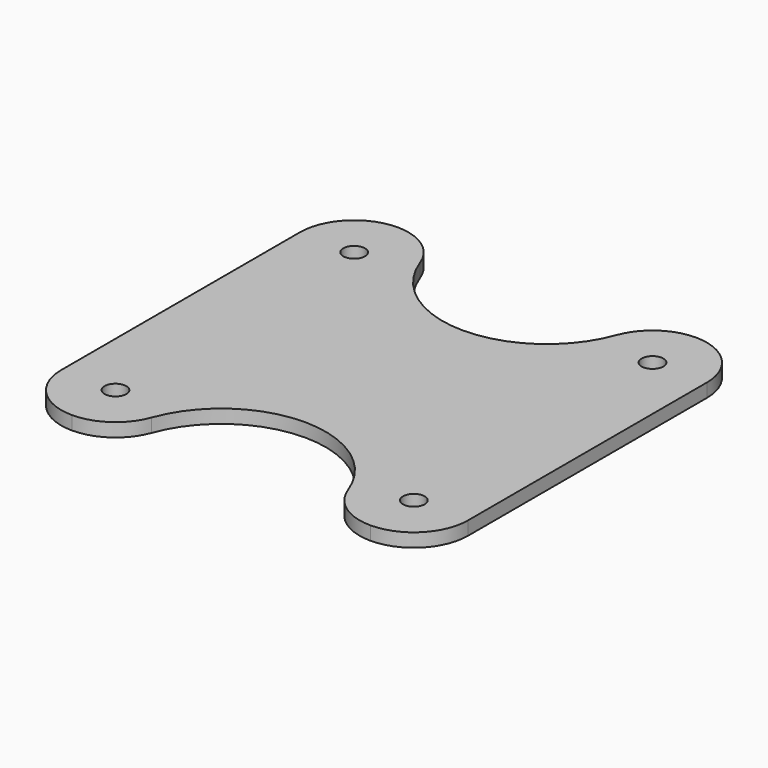
from build123d import *

# Parameters (mm, degrees)
F0_R     = 4
F1_DEPTH = 2.5
F2_R     = 20


with BuildPart() as f1:
    # F0 (on Top) → F1 (new body, symmetric)
    with BuildSketch(Plane.XY):
        with BuildLine():
            Line((38.5, -75), (75, -75))
            Line((75, -75), (75, 75))
            Line((75, 75), (38.5, 75))
            ThreePointArc((38.5, 75), (0, 36.5), (-38.5, 75))
            Line((-38.5, 75), (-75, 75))
            Line((-75, 75), (-75, -75))
            Line((-75, -75), (-38.5, -75))
            ThreePointArc((-38.5, -75), (0, -36.5), (38.5, -75))
        make_face()
        with Locations((-55, -55)):
            Circle(F0_R, mode=Mode.SUBTRACT)
        with Locations((55, -55)):
            Circle(F0_R, mode=Mode.SUBTRACT)
        with Locations((-55, 55)):
            Circle(F0_R, mode=Mode.SUBTRACT)
        with Locations((55, 55)):
            Circle(F0_R, mode=Mode.SUBTRACT)
    extrude(amount=F1_DEPTH, both=True)

    # F2
    f2_edges = [f1.edges().sort_by_distance(p)[0] for p in [
        (75, -75, 0),
        (75, 75, 0),
        (-75, 75, 0),
        (-38.5, 75, 0),
        (38.5, 75, 0),
        (-38.5, -75, 0),
        (38.5, -75, 0),
        (-75, -75, 0),
    ]]
    fillet(f2_edges, radius=F2_R)


solid = f1.part
